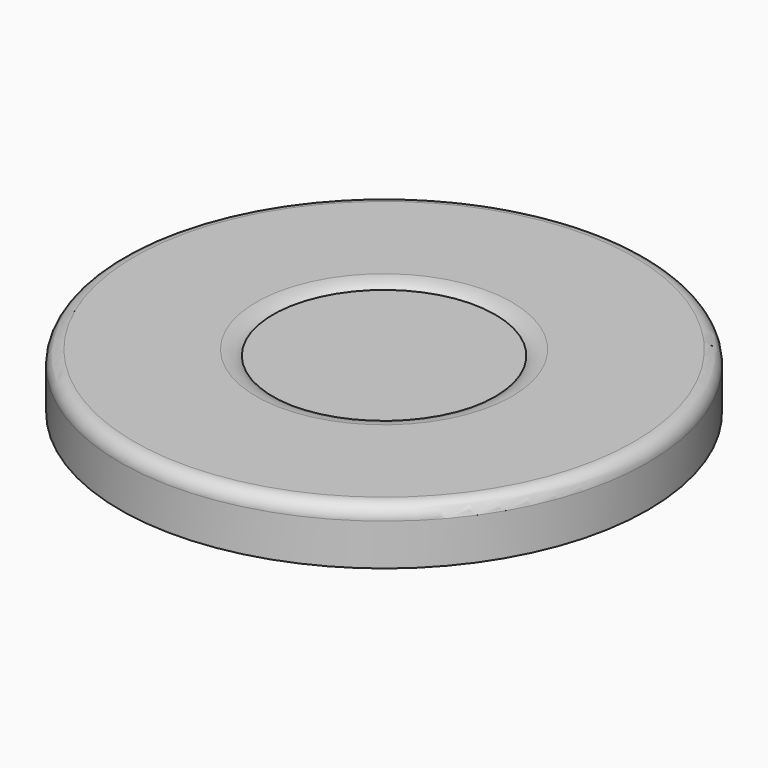
from build123d import *

# Parameters (mm, degrees)
F0_W   = 3.05
F0_H   = 0.4
F0_W_2 = 2.95
F0_H_2 = 2.5
F2_R   = 0.5


# Not quite as in the source:
# - a fillet or chamfer that OpenCascade refuses, or shapes differently, is made with other operations: its cross-section is extruded or revolved along the edge and cut away or added
# - a feature names something its author has since deleted; it is built from what else it names


with BuildPart() as f1:
    # F0 (on Front) → F1 (revolve)
    with BuildSketch(Plane.XZ):
        Polygon((0, 1.8), (0, 0), (3.05, 0), (6, 0), (9.5, 0), (9.5, 2), (4, 2), (4, 1.8), align=None)
        with Locations((1.525, -0.2)):
            Rectangle(F0_W, F0_H)
        with Locations((4.525, -0.2)):
            Rectangle(F0_W_2, F0_H)
        with Locations((1.525, -1.65)):
            Rectangle(F0_W, F0_H_2)
    revolve(axis=Axis((0, 0, 0.9), (0, 0, 1)))

    # F2
    f2_edges = [f1.edges().sort_by_distance(p)[0] for p in [
        (-9.5, 0, 2),
    ]]
    fillet(f2_edges, radius=F2_R)

    # F3: fillet of radius 1 on 1 edges, made by hand

    # F3_s1 → F3_t2 (revolve, cut)
    with BuildSketch(Plane.XZ):
        with BuildLine():
            ThreePointArc((4.6, 2), (4.283772234, 1.9486832981), (4, 1.8))
            Line((4, 1.8), (4, 2))
            Line((4, 2), (4.6, 2))
        make_face()
    revolve(axis=Axis((0, 0, 2), (0, 0, 1)), mode=Mode.SUBTRACT)


solid = f1.part
